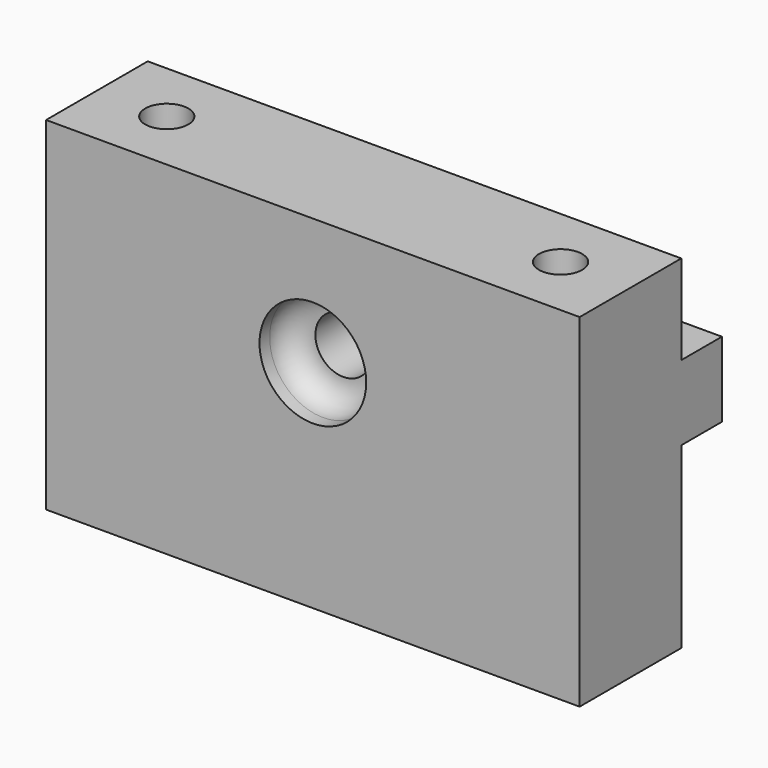
from build123d import *

# Parameters (mm, degrees)
F0_W     = 42
F0_H     = 10
F1_DEPTH = 27
F2_R     = 1.7
F3_DEPTH = 27.001
F4_W     = 13.5
F4_H     = 5.9
F5_DEPTH = 4
F4_R     = 2.2
F6_DEPTH = 25
F7_R     = 4.2
F8_DEPTH = 3
F9_R     = 1.99999


# Not quite as in the source:
# - a fillet or chamfer is up to 0.001 mm smaller than in the source, because OpenCascade refuses the exact size


with BuildPart() as f1:
    # F0 (on Top) → F1 (new body)
    with BuildSketch(Plane.XY):
        with Locations((4.146153807, 5)):
            Rectangle(F0_W, F0_H)
    extrude(amount=F1_DEPTH)

    # F2 (on face) → F3 (cut, through all)
    with BuildSketch(Plane.XY.offset(27)):
        with BuildLine():
            ThreePointArc((-13.053846193, 5), (-11.353846193, 3.3), (-9.653846193, 5))
            ThreePointArc((-9.653846193, 5), (-11.353846193, 6.7), (-13.053846193, 5))
        make_face()
        with Locations((19.646153807, 5)):
            Circle(F2_R)
    extrude(amount=-F3_DEPTH, mode=Mode.SUBTRACT)

    # F4 (on face) → F5 (join)
    with BuildSketch(Plane(origin=(0, 10, 0), x_dir=(-1, 0, 0), z_dir=(0, 1, 0))):
        with Locations((-18.396153807, 17)):
            Rectangle(F4_W, F4_H)
        with Locations((10.103846193, 17)):
            Rectangle(F4_W, F4_H)
    extrude(amount=F5_DEPTH)

    # F4 (on face) → F6 (cut)
    with BuildSketch(Plane(origin=(0, 10, 0), x_dir=(-1, 0, 0), z_dir=(0, 1, 0))):
        with Locations((-4.146153807, 17)):
            Circle(F4_R)
    extrude(amount=-F6_DEPTH, mode=Mode.SUBTRACT)

    # F7 (on face) → F8 (cut)
    with BuildSketch(Plane.XZ):
        with Locations((4.146153807, 17)):
            Circle(F7_R)
    extrude(amount=-F8_DEPTH, mode=Mode.SUBTRACT)

    # F9 (radius 2 in the source; OpenCascade refuses exactly that, so slightly less here)
    f9_edges = [f1.edges().sort_by_distance(p)[0] for p in [
        (-0.053846, 3, 17),
    ]]
    fillet(f9_edges, radius=F9_R)


solid = f1.part
